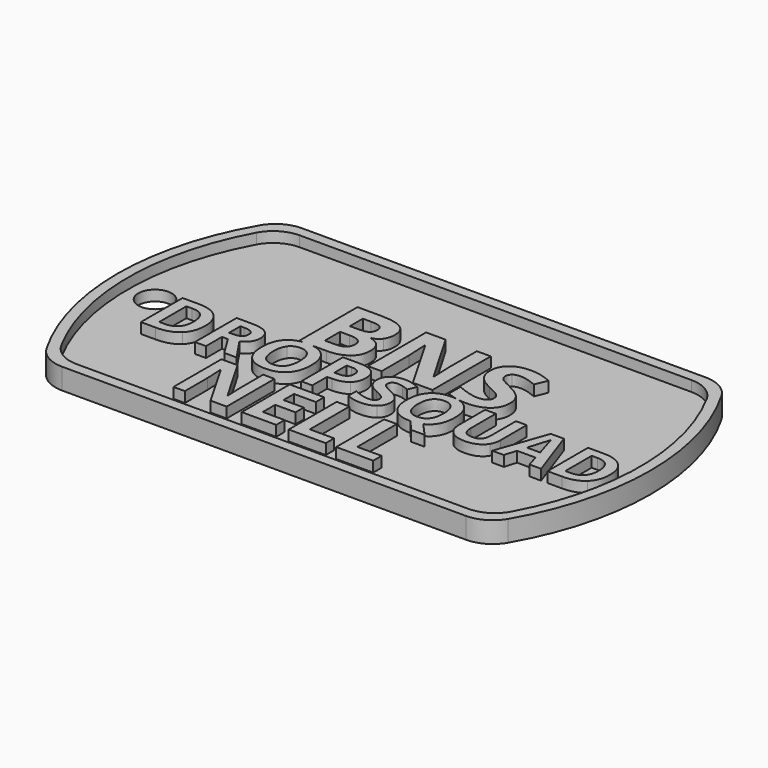
from build123d import *

# Parameters (mm, degrees)
F1_DEPTH     = 1
F3_DEPTH     = 1
F4_R         = 1.5875
F5_DEPTH     = 1
F6_TEXT_SIZE = 8.0000874328
F7_DEPTH     = 1


# Not quite as in the source:
# - Text() gives the source's letters only with a copy of the font that has no kerning and outlines rounded to 1/6400 em; it was checked with that copy


with BuildPart() as f1:
    # F0 (on Top) → F1 (new body)
    with BuildSketch(Plane.XY):
        with BuildLine():
            ThreePointArc((-19.2474145991, 14.2875), (-20.8349145991, 13.862130657), (-21.9970452561, 12.7))
            ThreePointArc((-21.9970452561, 12.7), (-25.4, 0), (-21.9970452561, -12.7))
            ThreePointArc((-21.9970452561, -12.7), (-20.8349145991, -13.862130657), (-19.2474145991, -14.2875))
            Line((-19.2474145991, -14.2875), (19.2474145991, -14.2875))
            ThreePointArc((19.2474145991, -14.2875), (20.8349145991, -13.862130657), (21.9970452561, -12.7))
            ThreePointArc((21.9970452561, -12.7), (25.4, 0), (21.9970452561, 12.7))
            ThreePointArc((21.9970452561, 12.7), (20.8349145991, 13.862130657), (19.2474145991, 14.2875))
            Line((19.2474145991, 14.2875), (-19.2474145991, 14.2875))
        make_face()
    extrude(amount=F1_DEPTH)

    # F2 (on face) → F3 (join)
    with BuildSketch(Plane.XY.offset(1)):
        with BuildLine():
            Line((19.2474145991, 14.2875), (-19.2474145991, 14.2875))
            ThreePointArc((-19.2474145991, 14.2875), (-20.8349145991, 13.862130657), (-21.9970452561, 12.7))
            ThreePointArc((-21.9970452561, 12.7), (-25.4, 0), (-21.9970452561, -12.7))
            ThreePointArc((-21.9970452561, -12.7), (-20.8349145991, -13.862130657), (-19.2474145991, -14.2875))
            Line((-19.2474145991, -14.2875), (19.2474145991, -14.2875))
            ThreePointArc((19.2474145991, -14.2875), (20.8349145991, -13.862130657), (21.9970452561, -12.7))
            ThreePointArc((21.9970452561, -12.7), (25.4, 0), (21.9970452561, 12.7))
            ThreePointArc((21.9970452561, 12.7), (20.8349145991, 13.862130657), (19.2474145991, 14.2875))
        make_face()
        with BuildLine():
            ThreePointArc((-21.4526124879, 11.6252061249), (-20.2856017842, 12.8404540819), (-18.6611352482, 13.2875))
            Line((-18.6611352482, 13.2875), (18.6611352482, 13.2875))
            ThreePointArc((18.6611352482, 13.2875), (20.2856017842, 12.8404540819), (21.4526124879, 11.6252061249))
            ThreePointArc((21.4526124879, 11.6252061249), (24.4, 0), (21.4526124879, -11.6252061249))
            ThreePointArc((21.4526124879, -11.6252061249), (20.2856017842, -12.8404540819), (18.6611352482, -13.2875))
            Line((18.6611352482, -13.2875), (-18.6611352482, -13.2875))
            ThreePointArc((-18.6611352482, -13.2875), (-20.2856017842, -12.8404540819), (-21.4526124879, -11.6252061249))
            ThreePointArc((-21.4526124879, -11.6252061249), (-24.4, 0), (-21.4526124879, 11.6252061249))
        make_face(mode=Mode.SUBTRACT)
    extrude(amount=F3_DEPTH)

    # F4 (on face) → F5 (cut)
    with BuildSketch(Plane.XY.offset(1)):
        with Locations((-21.821282804, 0)):
            Circle(F4_R)
    extrude(amount=-F5_DEPTH, mode=Mode.SUBTRACT)

    # F6 (on face) → F7 (join)
    with BuildSketch(Plane.XY.offset(1)):
        with BuildLine():
            Line((-5.9185070388, 6.9450069417), (-8.0799865466, 6.9450069417))
            Line((-8.0799865466, 6.9450069417), (-8.0799865466, 0))
            Line((-8.0799865466, 0), (-7.7755818095, 0))
            add(Edge.make_bspline(
                [(-7.7755818095, 0), (-7.5366505426, 0.0358699595), (-7.2685581615, 0.0358699595)],
                knots=[0.7657718145, 0.7657718145, 0.7657718145, 1, 1, 1], degree=2))
            add(Edge.make_bspline(
                [(-7.2685581615, 0.0358699595), (-7.0015731473, 0.0358699595), (-6.7638636977, 0)],
                knots=[0, 0, 0, 0.2332606961, 0.2332606961, 0.2332606961], degree=2))
            Line((-6.7638636977, 0), (-5.482259065, 0))
            add(Edge.make_bspline(
                [(-3.617184975, 0.5320097241), (-4.304237533, 0), (-5.482259065, 0)],
                knots=[0, 0, 0, 1, 1, 1], degree=2))
            add(Edge.make_bspline(
                [(-2.9301324169, 2.0140368128), (-2.9301324169, 1.0640194483), (-3.617184975, 0.5320097241)],
                knots=[0, 0, 0, 1, 1, 1], degree=2))
            add(Edge.make_bspline(
                [(-3.2227377652, 3.0879364417), (-2.9301324169, 2.6843690652), (-2.9301324169, 2.0140368128)],
                knots=[0, 0, 0, 1, 1, 1], degree=2))
            add(Edge.make_bspline(
                [(-4.1750351714, 3.6389465131), (-3.5153431135, 3.4915038181), (-3.2227377652, 3.0879364417)],
                knots=[0, 0, 0, 1, 1, 1], degree=2))
            Line((-4.1750351714, 3.6389465131), (-4.1750351714, 3.6860673744))
            add(Edge.make_bspline(
                [(-3.3983009742, 4.16563614), (-3.6901463085, 3.7666288469), (-4.1750351714, 3.6860673744)],
                knots=[0, 0, 0, 1, 1, 1], degree=2))
            add(Edge.make_bspline(
                [(-3.1064556398, 5.1878548242), (-3.1064556398, 4.5646434331), (-3.3983009742, 4.16563614)],
                knots=[0, 0, 0, 1, 1, 1], degree=2))
            add(Edge.make_bspline(
                [(-3.7737478366, 6.5247192596), (-3.1064556398, 6.1044315775), (-3.1064556398, 5.1878548242)],
                knots=[0, 0, 0, 1, 1, 1], degree=2))
            add(Edge.make_bspline(
                [(-5.9185070388, 6.9450069417), (-4.4410400335, 6.9450069417), (-3.7737478366, 6.5247192596)],
                knots=[0, 0, 0, 1, 1, 1], degree=2))
        make_face()
        with BuildLine():
            Line((-6.6070796246, 1.2160222266), (-6.6070796246, 3.0263753164))
            Line((-6.6070796246, 3.0263753164), (-5.6950629547, 3.0263753164))
            add(Edge.make_bspline(
                [(-4.4608003947, 2.1614795078), (-4.4608003947, 3.0263753164), (-5.6950629547, 3.0263753164)],
                knots=[0, 0, 0, 1, 1, 1], degree=2))
            add(Edge.make_bspline(
                [(-4.7503656874, 1.4485864774), (-4.4608003947, 1.6811507283), (-4.4608003947, 2.1614795078)],
                knots=[0, 0, 0, 1, 1, 1], degree=2))
            add(Edge.make_bspline(
                [(-5.6479420934, 1.2160222266), (-5.0399309801, 1.2160222266), (-4.7503656874, 1.4485864774)],
                knots=[0, 0, 0, 1, 1, 1], degree=2))
            Line((-5.6479420934, 1.2160222266), (-6.6070796246, 1.2160222266))
        make_face(mode=Mode.SUBTRACT)
        with BuildLine():
            Line((-5.7528240104, 4.193756654), (-6.6070796246, 4.193756654))
            Line((-6.6070796246, 4.193756654), (-6.6070796246, 5.7381048818))
            Line((-6.6070796246, 5.7381048818), (-5.8333854829, 5.7381048818))
            add(Edge.make_bspline(
                [(-4.9092085907, 5.5648217145), (-5.2010539251, 5.7381048818), (-5.8333854829, 5.7381048818)],
                knots=[0, 0, 0, 1, 1, 1], degree=2))
            add(Edge.make_bspline(
                [(-4.6173632563, 4.9917712402), (-4.6173632563, 5.3915385472), (-4.9092085907, 5.5648217145)],
                knots=[0, 0, 0, 1, 1, 1], degree=2))
            add(Edge.make_bspline(
                [(-4.8856481601, 4.3792000435), (-4.6173632563, 4.5646434331), (-4.6173632563, 4.9917712402)],
                knots=[0, 0, 0, 1, 1, 1], degree=2))
            add(Edge.make_bspline(
                [(-5.7528240104, 4.193756654), (-5.1539330638, 4.193756654), (-4.8856481601, 4.3792000435)],
                knots=[0, 0, 0, 1, 1, 1], degree=2))
        make_face(mode=Mode.SUBTRACT)
        with BuildLine():
            add(Edge.make_bspline(
                [(-7.7755818095, 0), (-7.5366505426, 0.0358699595), (-7.2685581615, 0.0358699595)],
                knots=[0.7657718145, 0.7657718145, 0.7657718145, 1, 1, 1], degree=2))
            Line((-7.7755818095, 0), (-6.7638636977, 0))
            add(Edge.make_bspline(
                [(-7.2685581615, 0.0358699595), (-7.0015731473, 0.0358699595), (-6.7638636977, 0)],
                knots=[0, 0, 0, 0.2332606961, 0.2332606961, 0.2332606961], degree=2))
        make_face()
        with BuildLine():
            Line((-6.7638636977, 0), (-7.7755818095, 0))
            add(Edge.make_bspline(
                [(-9.0261861781, -0.6179415754), (-8.5567296009, -0.11727113), (-7.7755818095, 0)],
                knots=[0, 0, 0, 0.7657718145, 0.7657718145, 0.7657718145], degree=2))
            add(Edge.make_bspline(
                [(-9.6392363954, -2.5119841351), (-9.6392363954, -1.2717531104), (-9.0261861781, -0.6179415754)],
                knots=[0, 0, 0, 1, 1, 1], degree=2))
            add(Edge.make_bspline(
                [(-9.0278166308, -4.4147224425), (-9.6392363954, -3.7522151598), (-9.6392363954, -2.5119841351)],
                knots=[0, 0, 0, 1, 1, 1], degree=2))
            add(Edge.make_bspline(
                [(-7.2750799723, -5.0772297252), (-8.4163968662, -5.0772297252), (-9.0278166308, -4.4147224425)],
                knots=[0, 0, 0, 1, 1, 1], degree=2))
            add(Edge.make_bspline(
                [(-5.5223433138, -4.4147224425), (-6.1337630784, -5.0772297252), (-7.2750799723, -5.0772297252)],
                knots=[0, 0, 0, 1, 1, 1], degree=2))
            add(Edge.make_bspline(
                [(-4.9109235492, -2.5185059459), (-4.9109235492, -3.7522151598), (-5.5223433138, -4.4147224425)],
                knots=[0, 0, 0, 1, 1, 1], degree=2))
            add(Edge.make_bspline(
                [(-5.5174519557, -0.6233764178), (-4.9109235492, -1.2826227951), (-4.9109235492, -2.5185059459)],
                knots=[0, 0, 0, 1, 1, 1], degree=2))
            add(Edge.make_bspline(
                [(-6.7638636977, 0), (-5.9825011239, -0.1179063094), (-5.5174519557, -0.6233764178)],
                knots=[0.2332606961, 0.2332606961, 0.2332606961, 1, 1, 1], degree=2))
        make_face()
        with BuildLine():
            add(Edge.make_bspline(
                [(-8.5348764295, -2.5185059459), (-8.5348764295, -3.3511237942), (-8.2191120889, -3.7723240765)],
                knots=[0, 0, 0, 1, 1, 1], degree=2))
            add(Edge.make_bspline(
                [(-8.2158511835, -1.2641443311), (-8.5348764295, -1.686975066), (-8.5348764295, -2.5185059459)],
                knots=[0, 0, 0, 1, 1, 1], degree=2))
            add(Edge.make_bspline(
                [(-7.2685581615, -0.8413135961), (-7.8968259374, -0.8413135961), (-8.2158511835, -1.2641443311)],
                knots=[0, 0, 0, 1, 1, 1], degree=2))
            add(Edge.make_bspline(
                [(-6.0152835152, -2.5185059459), (-6.0152835152, -0.8413135961), (-7.2685581615, -0.8413135961)],
                knots=[0, 0, 0, 1, 1, 1], degree=2))
            add(Edge.make_bspline(
                [(-7.2750799723, -4.1935243588), (-6.0152835152, -4.1935243588), (-6.0152835152, -2.5185059459)],
                knots=[0, 0, 0, 1, 1, 1], degree=2))
            add(Edge.make_bspline(
                [(-8.2191120889, -3.7723240765), (-7.9033477482, -4.1935243588), (-7.2750799723, -4.1935243588)],
                knots=[0, 0, 0, 1, 1, 1], degree=2))
        make_face(mode=Mode.SUBTRACT)
        with BuildLine():
            Line((2.7456513257, 0), (4.6168055269, 0))
            Line((4.6168055269, 0), (4.6168055269, 6.9450069417))
            Line((4.6168055269, 6.9450069417), (3.2913412999, 6.9450069417))
            Line((3.2913412999, 6.9450069417), (3.2913412999, 3.6571868465))
            add(Edge.make_bspline(
                [(3.3627826057, 1.7434718674), (3.2913412999, 3.0978166223), (3.2913412999, 3.6571868465)],
                knots=[0, 0, 0, 1, 1, 1], degree=2))
            Line((3.3627826057, 1.7434718674), (3.3293419945, 1.7434718674))
            Line((3.3293419945, 1.7434718674), (0.3136068725, 6.9450069417))
            Line((0.3136068725, 6.9450069417), (-1.5438670786, 6.9450069417))
            Line((-1.5438670786, 6.9450069417), (-1.5438670786, 0))
            Line((-1.5438670786, 0), (-0.2275230183, 0))
            Line((-0.2275230183, 0), (-0.2275230183, 3.268059734))
            add(Edge.make_bspline(
                [(-0.3187246853, 5.2532160189), (-0.2275230183, 3.8623905972), (-0.2275230183, 3.268059734)],
                knots=[0, 0, 0, 1, 1, 1], degree=2))
            Line((-0.3187246853, 5.2532160189), (-0.2761639074, 5.2532160189))
            Line((-0.2761639074, 5.2532160189), (2.7456513257, 0))
        make_face()
        with BuildLine():
            add(Edge.make_bspline(
                [(10.464352409, 1.9289152569), (10.464352409, 0.9880180591), (9.7871800316, 0.4461281544)],
                knots=[0, 0, 0, 1, 1, 1], degree=2))
            add(Edge.make_bspline(
                [(10.1033458105, 3.0757762194), (10.464352409, 2.6083676761), (10.464352409, 1.9289152569)],
                knots=[0, 0, 0, 1, 1, 1], degree=2))
            add(Edge.make_bspline(
                [(8.7680014029, 4.0098332922), (9.742339212, 3.5431847627), (10.1033458105, 3.0757762194)],
                knots=[0, 0, 0, 1, 1, 1], degree=2))
            add(Edge.make_bspline(
                [(7.8354643579, 4.4962421828), (8.0323079558, 4.3609597101), (8.7680014029, 4.0098332922)],
                knots=[0, 0, 0, 1, 1, 1], degree=2))
            add(Edge.make_bspline(
                [(7.5481791069, 4.7766873089), (7.63862076, 4.6315246556), (7.8354643579, 4.4962421828)],
                knots=[0, 0, 0, 1, 1, 1], degree=2))
            add(Edge.make_bspline(
                [(7.4577374538, 5.1164135184), (7.4577374538, 4.9218499622), (7.5481791069, 4.7766873089)],
                knots=[0, 0, 0, 1, 1, 1], degree=2))
            add(Edge.make_bspline(
                [(7.6811815379, 5.624102798), (7.4577374538, 5.4295392418), (7.4577374538, 5.1164135184)],
                knots=[0, 0, 0, 1, 1, 1], degree=2))
            add(Edge.make_bspline(
                [(8.3226332624, 5.8186663543), (7.9046256221, 5.8186663543), (7.6811815379, 5.624102798)],
                knots=[0, 0, 0, 1, 1, 1], degree=2))
            add(Edge.make_bspline(
                [(9.0370463206, 5.7282247012), (8.6737596804, 5.8186663543), (8.3226332624, 5.8186663543)],
                knots=[0, 0, 0, 1, 1, 1], degree=2))
            add(Edge.make_bspline(
                [(9.9566631294, 5.4097788806), (9.4003329608, 5.6377830481), (9.0370463206, 5.7282247012)],
                knots=[0, 0, 0, 1, 1, 1], degree=2))
            Line((9.9566631294, 5.4097788806), (10.4309117978, 6.5558798291))
            add(Edge.make_bspline(
                [(9.4026130024, 6.9161264138), (9.8943419903, 6.78844408), (10.4309117978, 6.5558798291)],
                knots=[0, 0, 0, 1, 1, 1], degree=2))
            add(Edge.make_bspline(
                [(8.3697541237, 7.0438087476), (8.9108840146, 7.0438087476), (9.4026130024, 6.9161264138)],
                knots=[0, 0, 0, 1, 1, 1], degree=2))
            add(Edge.make_bspline(
                [(6.643002562, 6.5171191207), (7.2677339809, 7.0438087476), (8.3697541237, 7.0438087476)],
                knots=[0, 0, 0, 1, 1, 1], degree=2))
            add(Edge.make_bspline(
                [(6.018271143, 5.0677726293), (6.018271143, 5.9904294938), (6.643002562, 6.5171191207)],
                knots=[0, 0, 0, 1, 1, 1], degree=2))
            add(Edge.make_bspline(
                [(6.208274616, 4.2135170152), (6.018271143, 4.5798437109), (6.018271143, 5.0677726293)],
                knots=[0, 0, 0, 1, 1, 1], degree=2))
            add(Edge.make_bspline(
                [(6.7167239094, 3.5720652906), (6.3982780889, 3.8471903194), (6.208274616, 4.2135170152)],
                knots=[0, 0, 0, 1, 1, 1], degree=2))
            add(Edge.make_bspline(
                [(7.6705413434, 2.9974947886), (7.03516973, 3.2969402619), (6.7167239094, 3.5720652906)],
                knots=[0, 0, 0, 1, 1, 1], degree=2))
            add(Edge.make_bspline(
                [(8.571157805, 2.5270461896), (8.3499937625, 2.6737288707), (7.6705413434, 2.9974947886)],
                knots=[0, 0, 0, 1, 1, 1], degree=2))
            add(Edge.make_bspline(
                [(8.9063239312, 2.2207605913), (8.7923218475, 2.3803635086), (8.571157805, 2.5270461896)],
                knots=[0, 0, 0, 1, 1, 1], degree=2))
            add(Edge.make_bspline(
                [(9.020326015, 1.8574739511), (9.020326015, 2.0611576741), (8.9063239312, 2.2207605913)],
                knots=[0, 0, 0, 1, 1, 1], degree=2))
            add(Edge.make_bspline(
                [(8.7611612779, 1.3064638797), (9.020326015, 1.4911472554), (9.020326015, 1.8574739511)],
                knots=[0, 0, 0, 1, 1, 1], degree=2))
            add(Edge.make_bspline(
                [(8.0186277058, 1.121780504), (8.5019965409, 1.121780504), (8.7611612779, 1.3064638797)],
                knots=[0, 0, 0, 1, 1, 1], degree=2))
            add(Edge.make_bspline(
                [(7.1271314109, 1.2494628378), (7.6143003155, 1.121780504), (8.0186277058, 1.121780504)],
                knots=[0, 0, 0, 1, 1, 1], degree=2))
            add(Edge.make_bspline(
                [(5.9377096705, 1.6917909228), (6.6399625064, 1.3771451716), (7.1271314109, 1.2494628378)],
                knots=[0, 0, 0, 1, 1, 1], degree=2))
            Line((5.9377096705, 1.6917909228), (5.9377096705, 0.3237659178))
            add(Edge.make_bspline(
                [(6.8880485788, 0.0025263686), (6.3784819127, 0.107301258), (5.9377096705, 0.3237659178)],
                knots=[0.4840276905, 0.4840276905, 0.4840276905, 1, 1, 1], degree=2))
            add(Edge.make_bspline(
                [(6.8880485788, 0.0025263686), (6.9892986218, -0.0121209069), (7.0851282227, -0.0334095928)],
                knots=[0.2246418033, 0.2246418033, 0.2246418033, 0.3264995474, 0.3264995474, 0.3264995474], degree=2))
            add(Edge.make_bspline(
                [(7.9046256221, -0.0957617503), (7.4756742652, -0.0957617503), (7.0851282227, -0.0334095928)],
                knots=[0, 0, 0, 0.3855186911, 0.3855186911, 0.3855186911], degree=2))
            add(Edge.make_bspline(
                [(9.7871800316, 0.4461281544), (9.1100076542, -0.0957617503), (7.9046256221, -0.0957617503)],
                knots=[0, 0, 0, 1, 1, 1], degree=2))
        make_face()
        with BuildLine():
            add(Edge.make_bspline(
                [(7.0851282227, -0.0334095928), (7.7187695833, -0.1741739475), (8.1154251048, -0.6053058002)],
                knots=[0.3264995474, 0.3264995474, 0.3264995474, 1, 1, 1], degree=2))
            add(Edge.make_bspline(
                [(7.0851282227, -0.0334095928), (6.985334618, -0.0174771652), (6.8880485788, 0.0025263686)],
                knots=[0.3855186911, 0.3855186911, 0.3855186911, 0.4840276905, 0.4840276905, 0.4840276905], degree=2))
            add(Edge.make_bspline(
                [(6.4150804769, 0.0348301507), (6.6647470275, 0.0348301507), (6.8880485788, 0.0025263686)],
                knots=[0, 0, 0, 0.2246418033, 0.2246418033, 0.2246418033], degree=2))
            add(Edge.make_bspline(
                [(4.7084030944, -0.6000285046), (5.303682033, 0.0348301507), (6.4150804769, 0.0348301507)],
                knots=[0, 0, 0, 1, 1, 1], degree=2))
            add(Edge.make_bspline(
                [(4.1131241557, -2.4391660056), (4.1131241557, -1.2348871599), (4.7084030944, -0.6000285046)],
                knots=[0, 0, 0, 1, 1, 1], degree=2))
            add(Edge.make_bspline(
                [(4.7068199057, -4.2867471795), (4.1131241557, -3.6434448513), (4.1131241557, -2.4391660056)],
                knots=[0, 0, 0, 1, 1, 1], degree=2))
            add(Edge.make_bspline(
                [(6.4087477222, -4.9300495077), (5.3005156556, -4.9300495077), (4.7068199057, -4.2867471795)],
                knots=[0, 0, 0, 1, 1, 1], degree=2))
            Line((6.4087477222, -4.9300495077), (6.4847407782, -4.9300495077))
            Line((6.4847407782, -4.9300495077), (7.3681600542, -6.0118950965))
            Line((7.3681600542, -6.0118950965), (8.677984811, -6.0118950965))
            Line((8.677984811, -6.0118950965), (7.5169797888, -4.714735849))
            add(Edge.make_bspline(
                [(8.402509983, -3.8724794784), (8.1006486772, -4.4477046939), (7.5169797888, -4.714735849)],
                knots=[0, 0, 0, 1, 1, 1], degree=2))
            add(Edge.make_bspline(
                [(8.7043712888, -2.4454987603), (8.7043712888, -3.2972542629), (8.402509983, -3.8724794784)],
                knots=[0, 0, 0, 1, 1, 1], degree=2))
            add(Edge.make_bspline(
                [(8.1154251048, -0.6053058002), (8.7043712888, -1.245441751), (8.7043712888, -2.4454987603)],
                knots=[0, 0, 0, 1, 1, 1], degree=2))
        make_face()
        with BuildLine():
            add(Edge.make_bspline(
                [(5.1854706125, -2.4454987603), (5.1854706125, -3.2539804393), (5.4920814843, -3.6629708449)],
                knots=[0, 0, 0, 1, 1, 1], degree=2))
            add(Edge.make_bspline(
                [(5.4952478616, -1.2274989461), (5.1854706125, -1.6380725403), (5.1854706125, -2.4454987603)],
                knots=[0, 0, 0, 1, 1, 1], degree=2))
            add(Edge.make_bspline(
                [(6.4150804769, -0.8169253519), (5.8050251107, -0.8169253519), (5.4952478616, -1.2274989461)],
                knots=[0, 0, 0, 1, 1, 1], degree=2))
            add(Edge.make_bspline(
                [(7.6320248319, -2.4454987603), (7.6320248319, -0.8169253519), (6.4150804769, -0.8169253519)],
                knots=[0, 0, 0, 1, 1, 1], degree=2))
            add(Edge.make_bspline(
                [(6.4087477222, -4.0719612504), (7.6320248319, -4.0719612504), (7.6320248319, -2.4454987603)],
                knots=[0, 0, 0, 1, 1, 1], degree=2))
            add(Edge.make_bspline(
                [(5.4920814843, -3.6629708449), (5.7986923561, -4.0719612504), (6.4087477222, -4.0719612504)],
                knots=[0, 0, 0, 1, 1, 1], degree=2))
        make_face(mode=Mode.SUBTRACT)
        with BuildLine():
            add(Edge.make_bspline(
                [(7.0851282227, -0.0334095928), (6.985334618, -0.0174771652), (6.8880485788, 0.0025263686)],
                knots=[0.3855186911, 0.3855186911, 0.3855186911, 0.4840276905, 0.4840276905, 0.4840276905], degree=2))
            add(Edge.make_bspline(
                [(6.8880485788, 0.0025263686), (6.9892986218, -0.0121209069), (7.0851282227, -0.0334095928)],
                knots=[0.2246418033, 0.2246418033, 0.2246418033, 0.3264995474, 0.3264995474, 0.3264995474], degree=2))
        make_face()
        with BuildLine():
            add(Edge.make_bspline(
                [(-15.0403827248, -2.4782881125), (-15.0403827248, -3.7043885471), (-15.738759967, -4.3565696293)],
                knots=[0, 0, 0, 1, 1, 1], degree=2))
            add(Edge.make_bspline(
                [(-15.713216208, -0.6842466521), (-15.0403827248, -1.3261015339), (-15.0403827248, -2.4782881125)],
                knots=[0, 0, 0, 1, 1, 1], degree=2))
            add(Edge.make_bspline(
                [(-17.6023674095, -0.0423917703), (-16.3860496912, -0.0423917703), (-15.713216208, -0.6842466521)],
                knots=[0, 0, 0, 1, 1, 1], degree=2))
            Line((-17.6023674095, -0.0423917703), (-19.1610801961, -0.0423917703))
            Line((-19.1610801961, -0.0423917703), (-19.1610801961, -5.0087507116))
            Line((-19.1610801961, -5.0087507116), (-17.7545429954, -5.0087507116))
            add(Edge.make_bspline(
                [(-15.738759967, -4.3565696293), (-16.4371372093, -5.0087507116), (-17.7545429954, -5.0087507116)],
                knots=[0, 0, 0, 1, 1, 1], degree=2))
        make_face()
        with BuildLine():
            add(Edge.make_bspline(
                [(-16.1349599745, -2.5054623243), (-16.1349599745, -0.9054447358), (-17.548018986, -0.9054447358)],
                knots=[0, 0, 0, 1, 1, 1], degree=2))
            add(Edge.make_bspline(
                [(-17.6567158331, -4.1391759353), (-16.1349599745, -4.1391759353), (-16.1349599745, -2.5054623243)],
                knots=[0, 0, 0, 1, 1, 1], degree=2))
            Line((-17.6567158331, -4.1391759353), (-18.1078077483, -4.1391759353))
            Line((-18.1078077483, -4.1391759353), (-18.1078077483, -0.9054447358))
            Line((-18.1078077483, -0.9054447358), (-17.548018986, -0.9054447358))
        make_face(mode=Mode.SUBTRACT)
        with BuildLine():
            Line((-12.9577511355, -5.0087507116), (-12.9577511355, -3.103294983))
            Line((-12.9577511355, -3.103294983), (-12.3979623733, -3.103294983))
            Line((-12.3979623733, -3.103294983), (-11.2120797721, -5.0087507116))
            Line((-11.2120797721, -5.0087507116), (-10.0435886664, -5.0087507116))
            add(Edge.make_bspline(
                [(-11.5044742906, -2.844596487), (-10.3827228292, -4.5196148999), (-10.0435886664, -5.0087507116)],
                knots=[0, 0, 0, 1, 1, 1], degree=2))
            add(Edge.make_bspline(
                [(-10.821314607, -2.3098079996), (-11.0620781232, -2.6511160993), (-11.5044742906, -2.844596487)],
                knots=[0, 0, 0, 1, 1, 1], degree=2))
            add(Edge.make_bspline(
                [(-10.5805510908, -1.5304516063), (-10.5805510908, -1.9684998999), (-10.821314607, -2.3098079996)],
                knots=[0, 0, 0, 1, 1, 1], degree=2))
            add(Edge.make_bspline(
                [(-11.0658825128, -0.4108740818), (-10.5805510908, -0.7793563933), (-10.5805510908, -1.5304516063)],
                knots=[0, 0, 0, 1, 1, 1], degree=2))
            add(Edge.make_bspline(
                [(-12.5642685493, -0.0423917703), (-11.5512139349, -0.0423917703), (-11.0658825128, -0.4108740818)],
                knots=[0, 0, 0, 1, 1, 1], degree=2))
            Line((-12.5642685493, -0.0423917703), (-14.0110235834, -0.0423917703))
            Line((-14.0110235834, -0.0423917703), (-14.0110235834, -5.0087507116))
            Line((-14.0110235834, -5.0087507116), (-12.9577511355, -5.0087507116))
        make_face()
        with BuildLine():
            Line((-12.6186169728, -2.2467638283), (-12.9577511355, -2.2467638283))
            Line((-12.9577511355, -2.2467638283), (-12.9577511355, -0.9054447358))
            Line((-12.9577511355, -0.9054447358), (-12.6381824053, -0.9054447358))
            add(Edge.make_bspline(
                [(-11.886543708, -1.0549029005), (-12.1294811611, -0.9054447358), (-12.6381824053, -0.9054447358)],
                knots=[0, 0, 0, 1, 1, 1], degree=2))
            add(Edge.make_bspline(
                [(-11.6436062548, -1.5576258181), (-11.6436062548, -1.2043610652), (-11.886543708, -1.0549029005)],
                knots=[0, 0, 0, 1, 1, 1], degree=2))
            add(Edge.make_bspline(
                [(-11.8811088656, -2.0804576523), (-11.6436062548, -1.9141514764), (-11.6436062548, -1.5576258181)],
                knots=[0, 0, 0, 1, 1, 1], degree=2))
            add(Edge.make_bspline(
                [(-12.6186169728, -2.2467638283), (-12.1186114764, -2.2467638283), (-11.8811088656, -2.0804576523)],
                knots=[0, 0, 0, 1, 1, 1], degree=2))
        make_face(mode=Mode.SUBTRACT)
        with BuildLine():
            add(Edge.make_bspline(
                [(-0.4510919152, -1.5913218407), (-0.4510919152, -2.3935045718), (-0.9521843801, -2.8179657595)],
                knots=[0, 0, 0, 1, 1, 1], degree=2))
            add(Edge.make_bspline(
                [(-0.9212057787, -0.4315264827), (-0.4510919152, -0.8206611951), (-0.4510919152, -1.5913218407)],
                knots=[0, 0, 0, 1, 1, 1], degree=2))
            add(Edge.make_bspline(
                [(-2.2956774095, -0.0423917703), (-1.3913196421, -0.0423917703), (-0.9212057787, -0.4315264827)],
                knots=[0, 0, 0, 1, 1, 1], degree=2))
            Line((-2.2956774095, -0.0423917703), (-3.8815644078, -0.0423917703))
            Line((-3.8815644078, -0.0423917703), (-3.8815644078, -5.0087507116))
            Line((-3.8815644078, -5.0087507116), (-2.82829196, -5.0087507116))
            Line((-2.82829196, -5.0087507116), (-2.82829196, -3.2424269472))
            Line((-2.82829196, -3.2424269472), (-2.3772000447, -3.2424269472))
            add(Edge.make_bspline(
                [(-0.9521843801, -2.8179657595), (-1.4532768449, -3.2424269472), (-2.3772000447, -3.2424269472)],
                knots=[0, 0, 0, 1, 1, 1], degree=2))
        make_face()
        with BuildLine():
            Line((-2.4815490179, -2.3793739817), (-2.82829196, -2.3793739817))
            Line((-2.82829196, -2.3793739817), (-2.82829196, -0.9054447358))
            Line((-2.82829196, -0.9054447358), (-2.350025833, -0.9054447358))
            add(Edge.make_bspline(
                [(-1.7163232147, -1.0820771123), (-1.9184993502, -0.9054447358), (-2.350025833, -0.9054447358)],
                knots=[0, 0, 0, 1, 1, 1], degree=2))
            add(Edge.make_bspline(
                [(-1.5141470793, -1.6293657371), (-1.5141470793, -1.2587094887), (-1.7163232147, -1.0820771123)],
                knots=[0, 0, 0, 1, 1, 1], degree=2))
            add(Edge.make_bspline(
                [(-1.7554540797, -2.1875240467), (-1.5141470793, -1.9956741116), (-1.5141470793, -1.6293657371)],
                knots=[0, 0, 0, 1, 1, 1], degree=2))
            add(Edge.make_bspline(
                [(-2.4815490179, -2.3793739817), (-1.9967610801, -2.3793739817), (-1.7554540797, -2.1875240467)],
                knots=[0, 0, 0, 1, 1, 1], degree=2))
        make_face(mode=Mode.SUBTRACT)
        with BuildLine():
            add(Edge.make_bspline(
                [(3.4534622113, -3.5241779718), (3.4534622113, -4.1775071615), (2.9832551774, -4.5537783346)],
                knots=[0, 0, 0, 1, 1, 1], degree=2))
            add(Edge.make_bspline(
                [(3.2027906725, -2.7278340725), (3.4534622113, -3.0523877491), (3.4534622113, -3.5241779718)],
                knots=[0, 0, 0, 1, 1, 1], degree=2))
            add(Edge.make_bspline(
                [(2.2755698434, -2.0792544488), (2.9521191336, -2.4032803958), (3.2027906725, -2.7278340725)],
                knots=[0, 0, 0, 1, 1, 1], degree=2))
            add(Edge.make_bspline(
                [(1.6280456788, -1.7415075332), (1.7647276337, -1.8354433941), (2.2755698434, -2.0792544488)],
                knots=[0, 0, 0, 1, 1, 1], degree=2))
            add(Edge.make_bspline(
                [(1.4285639068, -1.5467753272), (1.4913637239, -1.6475716723), (1.6280456788, -1.7415075332)],
                knots=[0, 0, 0, 1, 1, 1], degree=2))
            add(Edge.make_bspline(
                [(1.3657640897, -1.3108802159), (1.3657640897, -1.4459789821), (1.4285639068, -1.5467753272)],
                knots=[0, 0, 0, 1, 1, 1], degree=2))
            add(Edge.make_bspline(
                [(1.520916579, -0.9583568728), (1.3657640897, -1.093455639), (1.3657640897, -1.3108802159)],
                knots=[0, 0, 0, 1, 1, 1], degree=2))
            add(Edge.make_bspline(
                [(1.9663203239, -0.8232581066), (1.6760690683, -0.8232581066), (1.520916579, -0.9583568728)],
                knots=[0, 0, 0, 1, 1, 1], degree=2))
            add(Edge.make_bspline(
                [(2.4623861061, -0.8860579237), (2.2101313785, -0.8232581066), (1.9663203239, -0.8232581066)],
                knots=[0, 0, 0, 1, 1, 1], degree=2))
            add(Edge.make_bspline(
                [(3.1009388682, -1.1071766075), (2.7146408336, -0.9488577408), (2.4623861061, -0.8860579237)],
                knots=[0, 0, 0, 1, 1, 1], degree=2))
            Line((3.1009388682, -1.1071766075), (3.4302421109, -0.3113604378))
            add(Edge.make_bspline(
                [(2.7162240223, -0.0612166284), (3.0576650447, -0.1498751938), (3.4302421109, -0.3113604378)],
                knots=[0, 0, 0, 1, 1, 1], degree=2))
            add(Edge.make_bspline(
                [(1.9990395563, 0.0274419369), (2.3747829998, 0.0274419369), (2.7162240223, -0.0612166284)],
                knots=[0, 0, 0, 1, 1, 1], degree=2))
            add(Edge.make_bspline(
                [(0.8000380062, -0.3382746451), (1.2338317008, 0.0274419369), (1.9990395563, 0.0274419369)],
                knots=[0, 0, 0, 1, 1, 1], degree=2))
            add(Edge.make_bspline(
                [(0.3662443115, -1.3446549075), (0.3662443115, -0.7039912271), (0.8000380062, -0.3382746451)],
                knots=[0, 0, 0, 1, 1, 1], degree=2))
            add(Edge.make_bspline(
                [(0.4981767004, -1.9378229279), (0.3662443115, -1.6834572821), (0.3662443115, -1.3446549075)],
                knots=[0, 0, 0, 1, 1, 1], degree=2))
            add(Edge.make_bspline(
                [(0.8512277731, -2.3832266727), (0.6301090893, -2.1921885736), (0.4981767004, -1.9378229279)],
                knots=[0, 0, 0, 1, 1, 1], degree=2))
            add(Edge.make_bspline(
                [(1.5135283652, -2.7821902167), (1.0723464568, -2.5742647718), (0.8512277731, -2.3832266727)],
                knots=[0, 0, 0, 1, 1, 1], degree=2))
            add(Edge.make_bspline(
                [(2.1388878885, -3.1088548116), (1.9853185879, -3.0070030074), (1.5135283652, -2.7821902167)],
                knots=[0, 0, 0, 1, 1, 1], degree=2))
            add(Edge.make_bspline(
                [(2.3716166225, -3.3215298224), (2.2924571892, -3.2107066158), (2.1388878885, -3.1088548116)],
                knots=[0, 0, 0, 1, 1, 1], degree=2))
            add(Edge.make_bspline(
                [(2.4507760558, -3.57378455), (2.4507760558, -3.4323530291), (2.3716166225, -3.3215298224)],
                knots=[0, 0, 0, 1, 1, 1], degree=2))
            add(Edge.make_bspline(
                [(2.2708202774, -3.9563884777), (2.4507760558, -3.8281501957), (2.4507760558, -3.57378455)],
                knots=[0, 0, 0, 1, 1, 1], degree=2))
            add(Edge.make_bspline(
                [(1.7552285017, -4.0846267597), (2.090864499, -4.0846267597), (2.2708202774, -3.9563884777)],
                knots=[0, 0, 0, 1, 1, 1], degree=2))
            add(Edge.make_bspline(
                [(1.136201733, -3.9959681944), (1.4744763781, -4.0846267597), (1.7552285017, -4.0846267597)],
                knots=[0, 0, 0, 1, 1, 1], degree=2))
            add(Edge.make_bspline(
                [(0.3103049786, -3.6888295931), (0.7979270879, -3.9073096291), (1.136201733, -3.9959681944)],
                knots=[0, 0, 0, 1, 1, 1], degree=2))
            Line((0.3103049786, -3.6888295931), (0.3103049786, -4.638742793))
            add(Edge.make_bspline(
                [(1.6760690683, -4.9300495077), (0.9034729991, -4.9300495077), (0.3103049786, -4.638742793)],
                knots=[0, 0, 0, 1, 1, 1], degree=2))
            add(Edge.make_bspline(
                [(2.9832551774, -4.5537783346), (2.5130481434, -4.9300495077), (1.6760690683, -4.9300495077)],
                knots=[0, 0, 0, 1, 1, 1], degree=2))
        make_face()
        with BuildLine():
            Line((13.6291435009, -3.1611000376), (13.6291435009, -0.0411629053))
            Line((13.6291435009, -0.0411629053), (12.6095699996, -0.0411629053))
            Line((12.6095699996, -0.0411629053), (12.6095699996, -2.9869492842))
            add(Edge.make_bspline(
                [(12.3837017498, -3.8096796613), (12.6095699996, -3.5473980722), (12.6095699996, -2.9869492842)],
                knots=[0, 0, 0, 1, 1, 1], degree=2))
            add(Edge.make_bspline(
                [(11.6564904223, -4.0719612504), (12.1578335001, -4.0719612504), (12.3837017498, -3.8096796613)],
                knots=[0, 0, 0, 1, 1, 1], degree=2))
            add(Edge.make_bspline(
                [(10.9139749377, -3.81126285), (11.1382599988, -4.0719612504), (11.6564904223, -4.0719612504)],
                knots=[0, 0, 0, 1, 1, 1], degree=2))
            add(Edge.make_bspline(
                [(10.6896898766, -2.9932820389), (10.6896898766, -3.5505644495), (10.9139749377, -3.81126285)],
                knots=[0, 0, 0, 1, 1, 1], degree=2))
            Line((10.6896898766, -2.9932820389), (10.6896898766, -0.0411629053))
            Line((10.6896898766, -0.0411629053), (9.6711718345, -0.0411629053))
            Line((9.6711718345, -0.0411629053), (9.6711718345, -3.1484345282))
            add(Edge.make_bspline(
                [(10.1857081511, -4.4529819895), (9.6711718345, -3.9759144713), (9.6711718345, -3.1484345282)],
                knots=[0, 0, 0, 1, 1, 1], degree=2))
            add(Edge.make_bspline(
                [(11.6301039446, -4.9300495077), (10.7002444677, -4.9300495077), (10.1857081511, -4.4529819895)],
                knots=[0, 0, 0, 1, 1, 1], degree=2))
            add(Edge.make_bspline(
                [(12.6987562945, -4.7152635786), (12.2464920654, -4.9300495077), (11.6301039446, -4.9300495077)],
                knots=[0, 0, 0, 1, 1, 1], degree=2))
            add(Edge.make_bspline(
                [(13.3900820122, -4.0983477282), (13.1510205236, -4.5004776495), (12.6987562945, -4.7152635786)],
                knots=[0, 0, 0, 1, 1, 1], degree=2))
            add(Edge.make_bspline(
                [(13.6291435009, -3.1611000376), (13.6291435009, -3.6962178069), (13.3900820122, -4.0983477282)],
                knots=[0, 0, 0, 1, 1, 1], degree=2))
        make_face()
        Polygon((17.412964414, -3.7152160709), (17.7623213797, -4.8635555837), (18.8642206916, -4.8635555837), (17.1554323909, -0.0211091822), (15.9057688034, -0.0211091822), (14.2033132573, -4.8635555837), (15.3052125692, -4.8635555837), (15.654569535, -3.7152160709), align=None)
        with BuildLine():
            add(Edge.make_bspline(
                [(17.1680979002, -2.8581832727), (16.6836421682, -1.2982147066), (16.6224255398, -1.093455639)],
                knots=[0, 0, 0, 1, 1, 1], degree=2))
            Line((17.1680979002, -2.8581832727), (15.9121015581, -2.8581832727))
            add(Edge.make_bspline(
                [(16.5348224336, -0.7704851511), (16.4261101451, -1.1926687955), (15.9121015581, -2.8581832727)],
                knots=[0, 0, 0, 1, 1, 1], degree=2))
            add(Edge.make_bspline(
                [(16.6224255398, -1.093455639), (16.5612089113, -0.8886965715), (16.5348224336, -0.7704851511)],
                knots=[0, 0, 0, 1, 1, 1], degree=2))
        make_face(mode=Mode.SUBTRACT)
        with BuildLine():
            add(Edge.make_bspline(
                [(23.4723551704, -2.4064467732), (23.4723551704, -3.5970046504), (22.7942226916, -4.2302801171)],
                knots=[0, 0, 0, 1, 1, 1], degree=2))
            add(Edge.make_bspline(
                [(22.8190259807, -0.6644115104), (23.4723551704, -1.2876601155), (23.4723551704, -2.4064467732)],
                knots=[0, 0, 0, 1, 1, 1], degree=2))
            add(Edge.make_bspline(
                [(20.9846380457, -0.0411629053), (22.165696791, -0.0411629053), (22.8190259807, -0.6644115104)],
                knots=[0, 0, 0, 1, 1, 1], degree=2))
            Line((20.9846380457, -0.0411629053), (19.4711096805, -0.0411629053))
            Line((19.4711096805, -0.0411629053), (19.4711096805, -4.8635555837))
            Line((19.4711096805, -4.8635555837), (20.8368737702, -4.8635555837))
            add(Edge.make_bspline(
                [(22.7942226916, -4.2302801171), (22.1160902128, -4.8635555837), (20.8368737702, -4.8635555837)],
                knots=[0, 0, 0, 1, 1, 1], degree=2))
        make_face()
        with BuildLine():
            add(Edge.make_bspline(
                [(22.4095078456, -2.432833251), (22.4095078456, -0.8791974395), (21.0374110013, -0.8791974395)],
                knots=[0, 0, 0, 1, 1, 1], degree=2))
            add(Edge.make_bspline(
                [(20.9318650902, -4.0191882948), (22.4095078456, -4.0191882948), (22.4095078456, -2.432833251)],
                knots=[0, 0, 0, 1, 1, 1], degree=2))
            Line((20.9318650902, -4.0191882948), (20.4938495591, -4.0191882948))
            Line((20.4938495591, -4.0191882948), (20.4938495591, -0.8791974395))
            Line((20.4938495591, -0.8791974395), (21.0374110013, -0.8791974395))
        make_face(mode=Mode.SUBTRACT)
        with Locations((-11.4582274109, -11.6533078253)):
            Text('NELL', F6_TEXT_SIZE, font='Open Sans', font_style=FontStyle.BOLD, text_align=(TextAlign.LEFT, TextAlign.BOTTOM))
    extrude(amount=F7_DEPTH)


solid = f1.part
